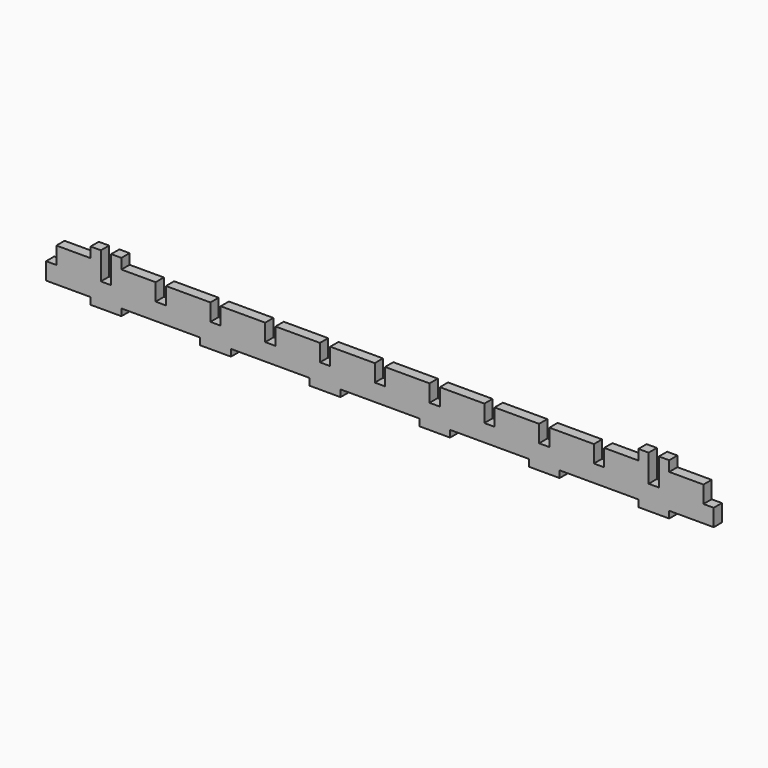
from build123d import *

# Parameters (mm, degrees)
F0_W     = 1.5
F0_H     = 5
F0_W_2   = 3
F0_H_2   = 2
F0_H_3   = 3
F1_DEPTH = 3


# Not quite as in the source:
# - a feature names something its author has since deleted; it is built from what else it names


with BuildPart() as f1:
    # F0 (on Front) → F1 (new body)
    with BuildSketch(Plane.XZ):
        with Locations((0.75, 2.5)):
            Rectangle(F0_W, F0_H)
        with Locations((-0.75, 2.5)):
            Rectangle(F0_W, F0_H)
        Polygon((1.5, 5), (1.5, 0), (11.5, 0), (14.5, 0), (14.5, 5), (14.5, 10), (11.5, 10), (1.5, 10), align=None)
        with Locations((13, -1)):
            Rectangle(F0_W_2, F0_H_2)
        with Locations((16, -1)):
            Rectangle(F0_W_2, F0_H_2)
        with Locations((16, 2.5)):
            Rectangle(F0_W_2, F0_H)
        with Locations((19, -1)):
            Rectangle(F0_W_2, F0_H_2)
        Polygon((17.5, 5), (17.5, 0), (20.5, 0), (30.5, 0), (30.5, 5), (30.5, 10), (20.5, 10), (17.5, 10), align=None)
        with Locations((13, 11.5)):
            Rectangle(F0_W_2, F0_H_3)
        with Locations((19, 11.5)):
            Rectangle(F0_W_2, F0_H_3)
        with Locations((32, 2.5)):
            Rectangle(F0_W_2, F0_H)
        Polygon((33.5, 5), (33.5, 0), (43.5, 0), (46.5, 0), (46.5, 5), (46.5, 10), (33.5, 10), align=None)
        with Locations((45, -1)):
            Rectangle(F0_W_2, F0_H_2)
        with Locations((48, -1)):
            Rectangle(F0_W_2, F0_H_2)
        with Locations((48, 2.5)):
            Rectangle(F0_W_2, F0_H)
        with Locations((51, -1)):
            Rectangle(F0_W_2, F0_H_2)
        Polygon((49.5, 5), (49.5, 0), (52.5, 0), (62.5, 0), (62.5, 5), (62.5, 10), (49.5, 10), align=None)
        with Locations((64, 2.5)):
            Rectangle(F0_W_2, F0_H)
        Polygon((78.5, 10), (65.5, 10), (65.5, 5), (65.5, 0), (75.5, 0), (78.5, 0), (78.5, 5), align=None)
        with Locations((77, -1)):
            Rectangle(F0_W_2, F0_H_2)
        Polygon((94.5, 10), (81.5, 10), (81.5, 5), (81.5, 0), (84.5, 0), (94.5, 0), (94.5, 5), align=None)
        with Locations((80, 2.5)):
            Rectangle(F0_W_2, F0_H)
        with Locations((80, -1)):
            Rectangle(F0_W_2, F0_H_2)
        with Locations((83, -1)):
            Rectangle(F0_W_2, F0_H_2)
        with Locations((95.25, 2.5)):
            Rectangle(F0_W, F0_H)
        with Locations((96.75, 2.5)):
            Rectangle(F0_W, F0_H)
        Polygon((110.5, 10), (97.5, 10), (97.5, 5), (97.5, 0), (107.5, 0), (110.5, 0), (110.5, 5), align=None)
        Polygon((126.5, 10), (113.5, 10), (113.5, 5), (113.5, 0), (116.5, 0), (126.5, 0), (126.5, 5), align=None)
        with Locations((112, 2.5)):
            Rectangle(F0_W_2, F0_H)
        with Locations((109, -1)):
            Rectangle(F0_W_2, F0_H_2)
        with Locations((112, -1)):
            Rectangle(F0_W_2, F0_H_2)
        with Locations((115, -1)):
            Rectangle(F0_W_2, F0_H_2)
        Polygon((142.5, 10), (129.5, 10), (129.5, 5), (129.5, 0), (139.5, 0), (142.5, 0), (142.5, 5), align=None)
        with Locations((128, 2.5)):
            Rectangle(F0_W_2, F0_H)
        Polygon((158.5, 10), (145.5, 10), (145.5, 5), (145.5, 0), (148.5, 0), (158.5, 0), (158.5, 5), align=None)
        with Locations((144, 2.5)):
            Rectangle(F0_W_2, F0_H)
        with Locations((144, -1)):
            Rectangle(F0_W_2, F0_H_2)
        with Locations((141, -1)):
            Rectangle(F0_W_2, F0_H_2)
        with Locations((147, -1)):
            Rectangle(F0_W_2, F0_H_2)
        with Locations((160, 2.5)):
            Rectangle(F0_W_2, F0_H)
        Polygon((171.5, 10), (161.5, 10), (161.5, 5), (161.5, 0), (171.5, 0), (174.5, 0), (174.5, 5), (174.5, 10), align=None)
        with Locations((173, 11.5)):
            Rectangle(F0_W_2, F0_H_3)
        with Locations((173, -1)):
            Rectangle(F0_W_2, F0_H_2)
        Polygon((180.5, 10), (177.5, 10), (177.5, 5), (177.5, 0), (180.5, 0), (190.5, 0), (190.5, 5), (190.5, 10), align=None)
        with Locations((179, 11.5)):
            Rectangle(F0_W_2, F0_H_3)
        with Locations((176, 2.5)):
            Rectangle(F0_W_2, F0_H)
        with Locations((176, -1)):
            Rectangle(F0_W_2, F0_H_2)
        with Locations((179, -1)):
            Rectangle(F0_W_2, F0_H_2)
        with Locations((191.25, 2.5)):
            Rectangle(F0_W, F0_H)
        with Locations((192.75, 2.5)):
            Rectangle(F0_W, F0_H)
    extrude(amount=F1_DEPTH)


solid = f1.part
